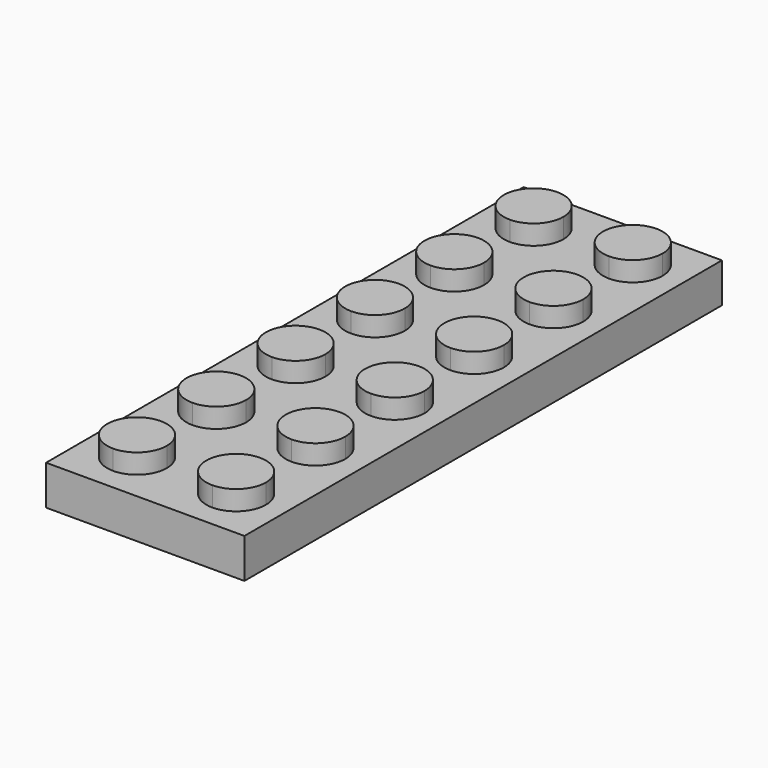
from build123d import *

# Parameters (mm, degrees)
F1_DEPTH = 3.175
F2_DEPTH = 4.7498
F3_T     = -1.6002


with BuildPart() as f1:
    # F0 (on Top) → F1 (new body)
    with BuildSketch(Plane.XY):
        with BuildLine():
            Line((5.7041967517, -35.7463070254), (9.6792967517, -35.7463070254))
            Line((9.6792967517, -35.7463070254), (9.6792967517, 12.1072929746))
            Line((9.6792967517, 12.1072929746), (5.7041967517, 12.1072929746))
            Line((5.7041967517, 12.1072929746), (5.7041967517, 10.5324929746))
            ThreePointArc((5.7041967517, 10.5324929746), (7.3924849024, 9.8331811253), (8.0917967517, 8.1448929746))
            ThreePointArc((8.0917967517, 8.1448929746), (7.3924849024, 6.4566048238), (5.7041967517, 5.7572929746))
            Line((5.7041967517, 5.7572929746), (5.7041967517, 2.5822929744))
            ThreePointArc((5.7041967517, 2.5822929744), (7.3924604194, 1.8829677352), (8.0917588785, 0.1946929747))
            ThreePointArc((8.0917588785, 0.1946929747), (7.3924604194, -1.4935817859), (5.7041967517, -2.192907025))
            Line((5.7041967517, -2.192907025), (5.7041967517, -5.3679070265))
            ThreePointArc((5.7041967517, -5.3679070265), (7.3924359362, -6.0672456551), (8.0917210053, -7.7555070253))
            ThreePointArc((8.0917210053, -7.7555070253), (7.3924359362, -9.4437683954), (5.7041967517, -10.143107024))
            Line((5.7041967517, -10.143107024), (5.7041967517, -13.3181070279))
            ThreePointArc((5.7041967517, -13.3181070279), (7.392411453, -14.0174590455), (8.0916831321, -15.7057070252))
            ThreePointArc((8.0916831321, -15.7057070252), (7.392411453, -17.3939550049), (5.7041967517, -18.0933070225))
            Line((5.7041967517, -18.0933070225), (5.7041967517, -21.2683070299))
            ThreePointArc((5.7041967517, -21.2683070299), (7.3923869696, -21.9676724359), (8.0916452589, -23.6559070251))
            ThreePointArc((8.0916452589, -23.6559070251), (7.3923869696, -25.3441416142), (5.7041967517, -26.0435070203))
            Line((5.7041967517, -26.0435070203), (5.7041967517, -29.2185070325))
            ThreePointArc((5.7041967517, -29.2185070325), (7.3923624861, -29.9178858265), (8.0916073858, -31.606107025))
            ThreePointArc((8.0916073858, -31.606107025), (7.3923624861, -33.2943282235), (5.7041967517, -33.9937070175))
            Line((5.7041967517, -33.9937070175), (5.7041967517, -35.7463070254))
        make_face()
        with BuildLine():
            Line((1.7290967517, -35.7463070254), (5.7041967517, -35.7463070254))
            Line((5.7041967517, -35.7463070254), (5.7041967517, -33.9937070175))
            ThreePointArc((5.7041967517, -33.9937070175), (3.3164073858, -31.606107025), (5.7041967517, -29.2185070325))
            Line((5.7041967517, -29.2185070325), (5.7041967517, -26.0435070203))
            ThreePointArc((5.7041967517, -26.0435070203), (3.3164452589, -23.6559070251), (5.7041967517, -21.2683070299))
            Line((5.7041967517, -21.2683070299), (5.7041967517, -18.0933070225))
            ThreePointArc((5.7041967517, -18.0933070225), (3.3164831321, -15.7057070252), (5.7041967517, -13.3181070279))
            Line((5.7041967517, -13.3181070279), (5.7041967517, -10.143107024))
            ThreePointArc((5.7041967517, -10.143107024), (3.3165210053, -7.7555070253), (5.7041967517, -5.3679070265))
            Line((5.7041967517, -5.3679070265), (5.7041967517, -2.192907025))
            ThreePointArc((5.7041967517, -2.192907025), (3.3165588785, 0.1946929747), (5.7041967517, 2.5822929744))
            Line((5.7041967517, 2.5822929744), (5.7041967517, 5.7572929746))
            ThreePointArc((5.7041967517, 5.7572929746), (3.3165967517, 8.1448929746), (5.7041967517, 10.5324929746))
            Line((5.7041967517, 10.5324929746), (5.7041967517, 12.1072929746))
            Line((5.7041967517, 12.1072929746), (1.7290967517, 12.1072929746))
            Line((1.7290967517, 12.1072929746), (-2.2460032483, 12.1072929746))
            Line((-2.2460032483, 12.1072929746), (-2.2460032483, 10.5324929746))
            ThreePointArc((-2.2460032483, 10.5324929746), (-0.5577150976, 9.8331811253), (0.1415967517, 8.1448929746))
            ThreePointArc((0.1415967517, 8.1448929746), (-0.5577150976, 6.4566048238), (-2.2460032483, 5.7572929746))
            Line((-2.2460032483, 5.7572929746), (-2.2460032483, 2.5822929744))
            ThreePointArc((-2.2460032483, 2.5822929744), (-0.5576906146, 1.8829945156), (0.1416346248, 0.1946929747))
            ThreePointArc((0.1416346248, 0.1946929747), (-0.5576906146, -1.4936085662), (-2.2460032483, -2.192907025))
            Line((-2.2460032483, -2.192907025), (-2.2460032483, -5.3679070265))
            ThreePointArc((-2.2460032483, -5.3679070265), (-0.5576661318, -6.0671920943), (0.141672498, -7.7555070253))
            ThreePointArc((0.141672498, -7.7555070253), (-0.5576661318, -9.4438219562), (-2.2460032483, -10.143107024))
            Line((-2.2460032483, -10.143107024), (-2.2460032483, -13.3181070279))
            ThreePointArc((-2.2460032483, -13.3181070279), (-0.5576416491, -14.0173787043), (0.1417103712, -15.7057070252))
            ThreePointArc((0.1417103712, -15.7057070252), (-0.5576416491, -17.394035346), (-2.2460032483, -18.0933070225))
            Line((-2.2460032483, -18.0933070225), (-2.2460032483, -21.2683070299))
            ThreePointArc((-2.2460032483, -21.2683070299), (-0.5576171665, -21.9675653144), (0.1417482444, -23.6559070251))
            ThreePointArc((0.1417482444, -23.6559070251), (-0.5576171665, -25.3442487357), (-2.2460032483, -26.0435070203))
            Line((-2.2460032483, -26.0435070203), (-2.2460032483, -29.2185070325))
            ThreePointArc((-2.2460032483, -29.2185070325), (-0.557592684, -29.9177519246), (0.1417861176, -31.606107025))
            ThreePointArc((0.1417861176, -31.606107025), (-0.557592684, -33.2944621254), (-2.2460032483, -33.9937070175))
            Line((-2.2460032483, -33.9937070175), (-2.2460032483, -35.7463070254))
            Line((-2.2460032483, -35.7463070254), (1.7290967517, -35.7463070254))
        make_face()
        with BuildLine():
            Line((-6.2211032483, -35.7463070254), (-2.2460032483, -35.7463070254))
            Line((-2.2460032483, -35.7463070254), (-2.2460032483, -33.9937070175))
            ThreePointArc((-2.2460032483, -33.9937070175), (-4.6334138824, -31.606107025), (-2.2460032483, -29.2185070325))
            Line((-2.2460032483, -29.2185070325), (-2.2460032483, -26.0435070203))
            ThreePointArc((-2.2460032483, -26.0435070203), (-4.6334517556, -23.6559070251), (-2.2460032483, -21.2683070299))
            Line((-2.2460032483, -21.2683070299), (-2.2460032483, -18.0933070225))
            ThreePointArc((-2.2460032483, -18.0933070225), (-4.6334896288, -15.7057070252), (-2.2460032483, -13.3181070279))
            Line((-2.2460032483, -13.3181070279), (-2.2460032483, -10.143107024))
            ThreePointArc((-2.2460032483, -10.143107024), (-4.633527502, -7.7555070253), (-2.2460032483, -5.3679070265))
            Line((-2.2460032483, -5.3679070265), (-2.2460032483, -2.192907025))
            ThreePointArc((-2.2460032483, -2.192907025), (-4.6335653752, 0.1946929747), (-2.2460032483, 2.5822929744))
            Line((-2.2460032483, 2.5822929744), (-2.2460032483, 5.7572929746))
            ThreePointArc((-2.2460032483, 5.7572929746), (-4.6336032483, 8.1448929746), (-2.2460032483, 10.5324929746))
            Line((-2.2460032483, 10.5324929746), (-2.2460032483, 12.1072929746))
            Line((-2.2460032483, 12.1072929746), (-6.2211032483, 12.1072929746))
            Line((-6.2211032483, 12.1072929746), (-6.2211032483, -35.7463070254))
        make_face()
    extrude(amount=F1_DEPTH)

    # F0 (on Top) → F2 (join)
    with BuildSketch(Plane.XY):
        with BuildLine():
            ThreePointArc((-2.2460032483, -29.2185070325), (-4.6334138824, -31.606107025), (-2.2460032483, -33.9937070175))
            Line((-2.2460032483, -33.9937070175), (-2.2460032483, -29.2185070325))
        make_face()
        with BuildLine():
            Line((-2.2460032483, -29.2185070325), (-2.2460032483, -33.9937070175))
            ThreePointArc((-2.2460032483, -33.9937070175), (-0.557592684, -33.2944621254), (0.1417861176, -31.606107025))
            ThreePointArc((0.1417861176, -31.606107025), (-0.557592684, -29.9177519246), (-2.2460032483, -29.2185070325))
        make_face()
        with BuildLine():
            ThreePointArc((-2.2460032483, -21.2683070299), (-4.6334517556, -23.6559070251), (-2.2460032483, -26.0435070203))
            Line((-2.2460032483, -26.0435070203), (-2.2460032483, -21.2683070299))
        make_face()
        with BuildLine():
            Line((-2.2460032483, -21.2683070299), (-2.2460032483, -26.0435070203))
            ThreePointArc((-2.2460032483, -26.0435070203), (-0.5576171665, -25.3442487357), (0.1417482444, -23.6559070251))
            ThreePointArc((0.1417482444, -23.6559070251), (-0.5576171665, -21.9675653144), (-2.2460032483, -21.2683070299))
        make_face()
        with BuildLine():
            ThreePointArc((-2.2460032483, -13.3181070279), (-4.6334896288, -15.7057070252), (-2.2460032483, -18.0933070225))
            Line((-2.2460032483, -18.0933070225), (-2.2460032483, -13.3181070279))
        make_face()
        with BuildLine():
            Line((-2.2460032483, -13.3181070279), (-2.2460032483, -18.0933070225))
            ThreePointArc((-2.2460032483, -18.0933070225), (-0.5576416491, -17.394035346), (0.1417103712, -15.7057070252))
            ThreePointArc((0.1417103712, -15.7057070252), (-0.5576416491, -14.0173787043), (-2.2460032483, -13.3181070279))
        make_face()
        with BuildLine():
            Line((-2.2460032483, -10.143107024), (-2.2460032483, -5.3679070265))
            ThreePointArc((-2.2460032483, -5.3679070265), (-4.633527502, -7.7555070253), (-2.2460032483, -10.143107024))
        make_face()
        with BuildLine():
            ThreePointArc((0.141672498, -7.7555070253), (-0.5576661318, -6.0671920943), (-2.2460032483, -5.3679070265))
            Line((-2.2460032483, -5.3679070265), (-2.2460032483, -10.143107024))
            ThreePointArc((-2.2460032483, -10.143107024), (-0.5576661318, -9.4438219562), (0.141672498, -7.7555070253))
        make_face()
        with BuildLine():
            Line((-2.2460032483, -2.192907025), (-2.2460032483, 2.5822929744))
            ThreePointArc((-2.2460032483, 2.5822929744), (-4.6335653752, 0.1946929747), (-2.2460032483, -2.192907025))
        make_face()
        with BuildLine():
            ThreePointArc((0.1416346248, 0.1946929747), (-0.5576906146, 1.8829945156), (-2.2460032483, 2.5822929744))
            Line((-2.2460032483, 2.5822929744), (-2.2460032483, -2.192907025))
            ThreePointArc((-2.2460032483, -2.192907025), (-0.5576906146, -1.4936085662), (0.1416346248, 0.1946929747))
        make_face()
        with BuildLine():
            Line((-2.2460032483, 5.7572929746), (-2.2460032483, 10.5324929746))
            ThreePointArc((-2.2460032483, 10.5324929746), (-4.6336032483, 8.1448929746), (-2.2460032483, 5.7572929746))
        make_face()
        with BuildLine():
            ThreePointArc((0.1415967517, 8.1448929746), (-0.5577150976, 9.8331811253), (-2.2460032483, 10.5324929746))
            Line((-2.2460032483, 10.5324929746), (-2.2460032483, 5.7572929746))
            ThreePointArc((-2.2460032483, 5.7572929746), (-0.5577150976, 6.4566048238), (0.1415967517, 8.1448929746))
        make_face()
        with BuildLine():
            ThreePointArc((5.7041967517, -29.2185070325), (3.3164073858, -31.606107025), (5.7041967517, -33.9937070175))
            Line((5.7041967517, -33.9937070175), (5.7041967517, -29.2185070325))
        make_face()
        with BuildLine():
            Line((5.7041967517, -29.2185070325), (5.7041967517, -33.9937070175))
            ThreePointArc((5.7041967517, -33.9937070175), (7.3923624861, -33.2943282235), (8.0916073858, -31.606107025))
            ThreePointArc((8.0916073858, -31.606107025), (7.3923624861, -29.9178858265), (5.7041967517, -29.2185070325))
        make_face()
        with BuildLine():
            ThreePointArc((5.7041967517, -21.2683070299), (3.3164452589, -23.6559070251), (5.7041967517, -26.0435070203))
            Line((5.7041967517, -26.0435070203), (5.7041967517, -21.2683070299))
        make_face()
        with BuildLine():
            Line((5.7041967517, -21.2683070299), (5.7041967517, -26.0435070203))
            ThreePointArc((5.7041967517, -26.0435070203), (7.3923869696, -25.3441416142), (8.0916452589, -23.6559070251))
            ThreePointArc((8.0916452589, -23.6559070251), (7.3923869696, -21.9676724359), (5.7041967517, -21.2683070299))
        make_face()
        with BuildLine():
            ThreePointArc((5.7041967517, -13.3181070279), (3.3164831321, -15.7057070252), (5.7041967517, -18.0933070225))
            Line((5.7041967517, -18.0933070225), (5.7041967517, -13.3181070279))
        make_face()
        with BuildLine():
            Line((5.7041967517, -10.143107024), (5.7041967517, -5.3679070265))
            ThreePointArc((5.7041967517, -5.3679070265), (3.3165210053, -7.7555070253), (5.7041967517, -10.143107024))
        make_face()
        with BuildLine():
            ThreePointArc((8.0917210053, -7.7555070253), (7.3924359362, -6.0672456551), (5.7041967517, -5.3679070265))
            Line((5.7041967517, -5.3679070265), (5.7041967517, -10.143107024))
            ThreePointArc((5.7041967517, -10.143107024), (7.3924359362, -9.4437683954), (8.0917210053, -7.7555070253))
        make_face()
        with BuildLine():
            Line((5.7041967517, -13.3181070279), (5.7041967517, -18.0933070225))
            ThreePointArc((5.7041967517, -18.0933070225), (7.392411453, -17.3939550049), (8.0916831321, -15.7057070252))
            ThreePointArc((8.0916831321, -15.7057070252), (7.392411453, -14.0174590455), (5.7041967517, -13.3181070279))
        make_face()
        with BuildLine():
            Line((5.7041967517, -2.192907025), (5.7041967517, 2.5822929744))
            ThreePointArc((5.7041967517, 2.5822929744), (3.3165588785, 0.1946929747), (5.7041967517, -2.192907025))
        make_face()
        with BuildLine():
            ThreePointArc((8.0917588785, 0.1946929747), (7.3924604194, 1.8829677352), (5.7041967517, 2.5822929744))
            Line((5.7041967517, 2.5822929744), (5.7041967517, -2.192907025))
            ThreePointArc((5.7041967517, -2.192907025), (7.3924604194, -1.4935817859), (8.0917588785, 0.1946929747))
        make_face()
        with BuildLine():
            Line((5.7041967517, 5.7572929746), (5.7041967517, 10.5324929746))
            ThreePointArc((5.7041967517, 10.5324929746), (3.3165967517, 8.1448929746), (5.7041967517, 5.7572929746))
        make_face()
        with BuildLine():
            ThreePointArc((8.0917967517, 8.1448929746), (7.3924849024, 9.8331811253), (5.7041967517, 10.5324929746))
            Line((5.7041967517, 10.5324929746), (5.7041967517, 5.7572929746))
            ThreePointArc((5.7041967517, 5.7572929746), (7.3924849024, 6.4566048238), (8.0917967517, 8.1448929746))
        make_face()
    extrude(amount=F2_DEPTH)

    # F3
    f3_openings = [f1.faces().sort_by_distance(p)[0] for p in [
        (1.729097, -11.819507, 0),
    ]]
    offset(amount=F3_T, openings=f3_openings, kind=Kind.INTERSECTION)


solid = f1.part
